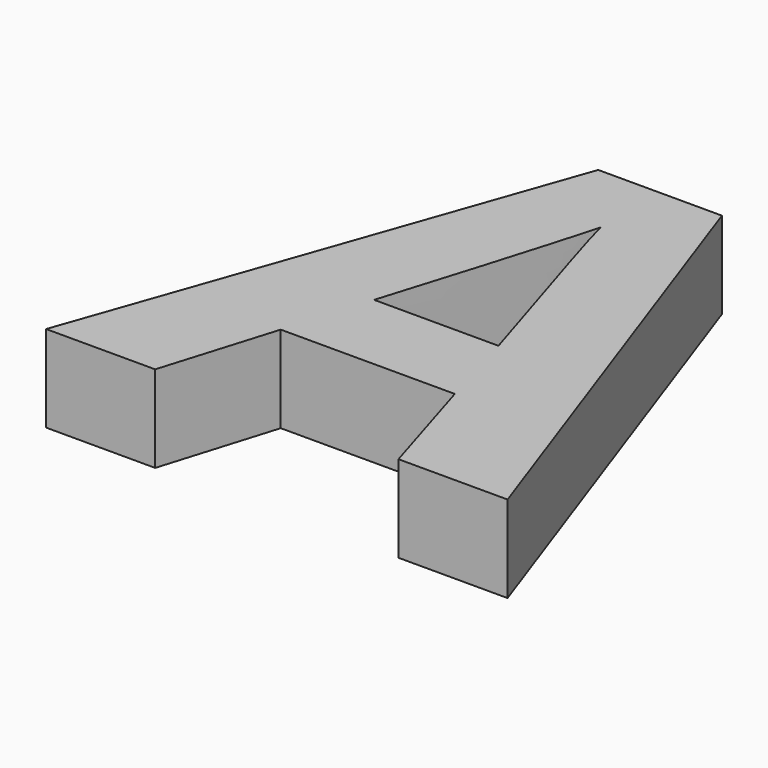
from build123d import *

# Parameters (mm, degrees)
F0_TEXT_SIZE = 77.0596580373
F1_DEPTH     = 10


# Not quite as in the source:
# - Text() gives the source's letters only with a copy of the font that has no kerning and outlines rounded to 1/6400 em; it was checked with that copy


with BuildPart() as f1:
    # F0 (on Top) → F1 (new body)
    with BuildSketch(Plane.XY):
        with Locations((0, 0)):
            Text('A', F0_TEXT_SIZE, font='Open Sans', font_style=FontStyle.BOLD, text_align=(TextAlign.LEFT, TextAlign.BOTTOM))
    extrude(amount=F1_DEPTH)


solid = f1.part
